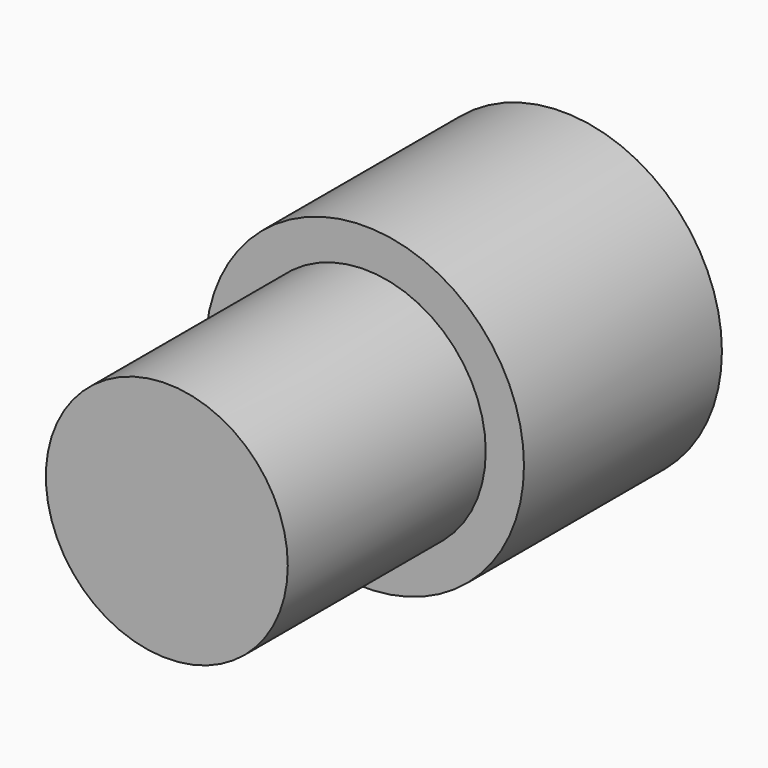
from build123d import *

# Parameters (mm, degrees)
F0_R     = 49.0283190444
F1_DEPTH = 76.2
F2_R     = 37.255304708
F3_DEPTH = 152.4
F4_R     = 23.611936081
F5_DEPTH = 273


# Not quite as in the source:
# - an extrude ends at something that could not be found from the text; its depth is read off the source's solid


with BuildPart() as f1:
    # F0 (on Front) → F1 (new body)
    with BuildSketch(Plane.XZ):
        Circle(F0_R)
    extrude(amount=F1_DEPTH)

    # F2 (on Front) → F3 (join)
    with BuildSketch(Plane.XZ):
        Circle(F2_R)
    extrude(amount=F3_DEPTH)

    # F4 (on Front) → F5 (cut, through all)
    with BuildSketch(Plane.XZ):
        Circle(F4_R)
    extrude(amount=-F5_DEPTH, mode=Mode.SUBTRACT)


solid = f1.part
